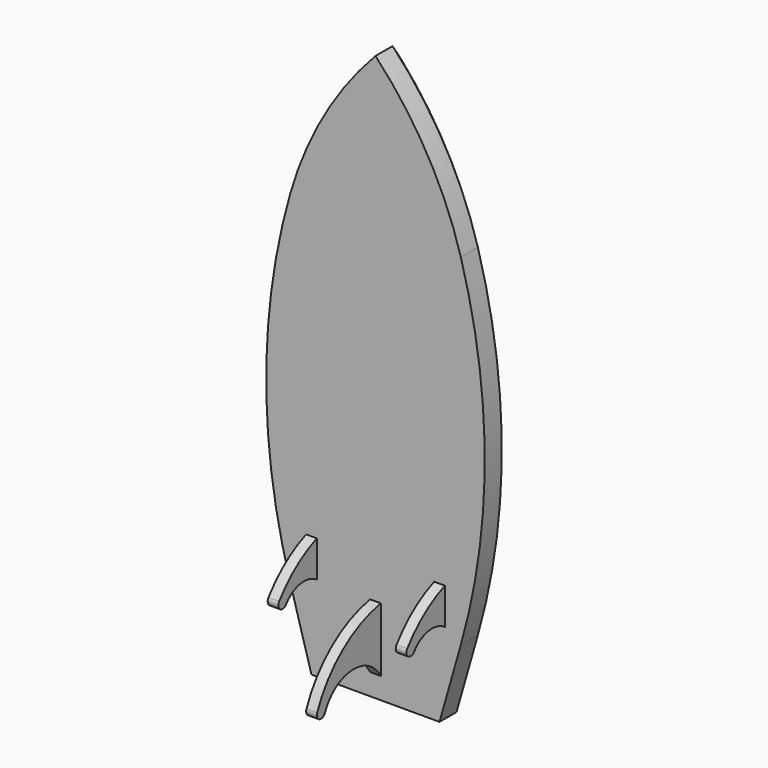
from build123d import *

# Parameters (mm, degrees)
F1_DEPTH = 4.7625
F3_DEPTH = 0.79375
F6_DEPTH = 0.79375
F7_SIZE  = 1.5875
F9_DEPTH = 1.5875


# Not quite as in the source:
# - a pattern or mirror of a feature is missing from the dataset's text; its kind, count and spacing are read off the source's solid


with BuildPart() as f1:
    # F0 (on Front) → F1 (new body)
    with BuildSketch(Plane.XZ):
        with BuildLine():
            Line((-12.7, 0), (-9.525, -11.1125))
            Line((-9.525, -11.1125), (0, -11.1125))
            Line((0, -11.1125), (9.525, -11.1125))
            Line((9.525, -11.1125), (12.7, 0))
            ThreePointArc((12.7, 0), (16.2573955939, 25.4), (12.7, 50.8))
            ThreePointArc((12.7, 50.8), (7.6947096259, 62.6809055005), (0, 73.025))
            ThreePointArc((0, 73.025), (-7.6947096259, 62.6809055005), (-12.7, 50.8))
            ThreePointArc((-12.7, 50.8), (-16.2573955939, 25.4), (-12.7, 0))
        make_face()
    extrude(amount=F1_DEPTH)

    # F2 (on Right) → F3 (join, symmetric)
    with BuildSketch(Plane.YZ):
        with BuildLine():
            Line((-4.7625, -7.9375), (-4.7625, 1.5875))
            ThreePointArc((-4.7625, 1.5875), (-11.8992437218, -1.6651672616), (-16.6078313322, -7.9375))
            ThreePointArc((-16.6078313322, -7.9375), (-16.1799545886, -8.9752859207), (-15.1421686678, -8.5474091771))
            ThreePointArc((-15.1421686678, -8.5474091771), (-10.143051775, -4.9967519132), (-4.7625, -7.9375))
        make_face()
    extrude(amount=F3_DEPTH, both=True)

    # F5 (on offset) → F6 (join, symmetric)
    with BuildSketch(Plane.YZ.offset(9.525)):
        with BuildLine():
            Line((-4.7625, 1.5875), (-4.7625, 6.9977))
            ThreePointArc((-4.7625, 6.9977), (-8.6423632972, 4.7890693745), (-11.7538487922, 1.5875))
            ThreePointArc((-11.7538487922, 1.5875), (-11.5801652534, 0.4784859544), (-10.4711512078, 0.6521694931))
            ThreePointArc((-10.4711512078, 0.6521694931), (-7.8086096464, 2.2903602428), (-4.7625, 1.5875))
        make_face()
    f6 = extrude(amount=F6_DEPTH, both=True)

    # F6_copies: F6 across plane
    add(f6.mirror(Plane(origin=(0, 0, 0), x_dir=(0, 0, -1), z_dir=(-1, 0, 0))))

    # F7
    f7_edges = [f1.edges().sort_by_distance(p)[0] for p in [
        (-16.257396, 0, 25.4),
        (16.257396, 0, 25.4),
        (0, 0, -11.1125),
        (-11.1125, 0, -5.55625),
        (11.1125, 0, -5.55625),
        (7.69471, 0, 62.680906),
        (-7.69471, 0, 62.680906),
    ]]
    chamfer(f7_edges, length=F7_SIZE)

    # F8 (on face) → F9 (cut)
    with BuildSketch(Plane(origin=(0, 0, 0), x_dir=(-1, 0, 0), z_dir=(0, 1, 0))):
        Polygon((-6.6182743758, 28.1248632818), (-6.6700917669, 25.4352521151), (4.5057865791, 25.4352521151), (4.5057865791, 28.058398515), (2.0293486305, 28.058398515), (0.9048542867, 29.1962967539), (4.5085526071, 31.6355861723), (4.5085526071, 34.4496265318), (-0.5952421925, 30.9949442744), (-3.6387769505, 33.8591597974), (-3.6387769505, 30.7964850217), (-1.2080913875, 28.5090107937), (-1.2080913875, 28.1248632818), align=None)
        with BuildLine():
            Line((0.4666208988, 17.5453214468), (-3.6424577702, 17.5453214468))
            Line((-3.6424577702, 17.5453214468), (-3.6424577702, 14.9797564372))
            Line((-3.6424577702, 14.9797564372), (0.4666208988, 14.9797564372))
            ThreePointArc((0.4666208988, 14.9797564372), (4.6440088446, 19.157144383), (0.4666208988, 23.3345323288))
            Line((0.4666208988, 23.3345323288), (-3.6424577702, 23.3345323288))
            Line((-3.6424577702, 23.3345323288), (-3.6424577702, 20.7669679075))
            Line((-3.6424577702, 20.7669679075), (0.4666208988, 20.7669679075))
            ThreePointArc((0.4666208988, 20.7669679075), (2.0774441292, 19.1561446772), (0.4666208988, 17.5453214468))
        make_face()
        with BuildLine():
            Line((8.6546270177, 44.8338016868), (6.6723674536, 44.8338016868))
            add(Edge.make_bspline(
                [(-4.5172106475, 2.828539582), (-4.2102957065, 2.1494447633), (-3.6325259568, 0.8710435159), (-2.8108192248, -0.6144651088), (-1.8892552518, -1.6043922723), (-1.0524312759, -2.1879868929), (-0.1957544902, -2.506421982), (0.7811404131, -2.2568299422), (1.5879280313, -1.7739319167), (2.1757138001, -1.1453271009), (2.6284881315, -0.4594989905), (3.409904115, 0.8193268379), (4.0612270575, 2.2527381247), (5.1265355245, 5.1336336674), (5.8584252285, 8.1588665014), (6.6285848683, 12.0725691399), (7.1356428748, 15.4950302956), (7.4330256401, 19.1136138456), (7.6363893931, 21.7933478819), (7.7823315333, 24.9471808649), (7.8520468643, 29.2726933395), (7.7372059862, 32.0576492162), (7.7120020586, 34.9143380941), (7.4839798645, 37.6447246054), (7.3090766206, 40.0269481522), (6.9398489174, 42.6509249895), (6.7587947507, 44.1284812873), (6.6723674536, 44.8338016868)],
                knots=[0, 0, 0, 0, 0.0403691258, 0.0759951914, 0.1074815982, 0.1348944717, 0.1603897512, 0.1873090479, 0.2138867667, 0.2387664663, 0.263585301, 0.2963900232, 0.3311454371, 0.3784414378, 0.4275924791, 0.4818900852, 0.5334929951, 0.5852044455, 0.629771183, 0.6785525678, 0.7354652809, 0.7815573057, 0.8274001502, 0.8726253751, 0.9150940097, 0.9594696141, 1, 1, 1, 1], degree=3))
            ThreePointArc((-4.5172106475, 2.828539582), (-5.0858860374, 2.569399443), (-5.7084131986, 2.5145793334))
            add(Edge.make_bspline(
                [(-5.7084131986, 2.5145793334), (-5.506614464, 2.0648957392), (-5.0657293675, 1.0824376715), (-3.9032511452, -0.8031134896), (-2.9635999986, -1.8497808999), (-1.9867636738, -2.5987631458), (-0.8338053387, -3.0579918443), (-0.0168141797, -3.2294336457), (0.8209716365, -3.0655957536), (1.5138835925, -2.8005151737), (2.3358805397, -2.394543116), (3.2541179547, -1.5281590897), (4.1857809915, -0.4409412593), (5.176415684, 1.2296860629), (6.2809613816, 3.4291719671), (6.9421799555, 5.2390225088), (7.6342063093, 7.5576057945), (8.099356579, 9.4090035643), (8.7001521406, 12.0174155991), (9.1556024302, 14.8338769341), (9.5981195448, 17.6634096123), (9.8314203891, 20.6701764069), (10.0211103061, 24.1869823425), (10.1148431942, 26.2740195603), (10.1813479944, 28.5970208607), (10.0793257033, 30.7502618751), (10.0643211933, 33.23997833), (9.8679121246, 36.2080072223), (9.5625129269, 39.346165649), (9.2718834561, 42.0400533513), (8.8620401687, 43.8950344105), (8.6546270177, 44.8338016868)],
                knots=[0, 0, 0, 0, 0.0307215617, 0.0671197405, 0.0962538158, 0.1231797002, 0.1502640042, 0.1725469817, 0.1946999143, 0.2157414832, 0.2389236845, 0.2662186517, 0.2954186022, 0.3296826311, 0.3680005184, 0.4024574657, 0.4400039897, 0.4741040733, 0.5138479488, 0.555501876, 0.5966862081, 0.6397342099, 0.6854696479, 0.7211558824, 0.7579160018, 0.7939211093, 0.8323591282, 0.8748241347, 0.9183554421, 0.9586813898, 1, 1, 1, 1], degree=3))
        make_face()
        with BuildLine():
            Line((0.5082425971, 38.120555704), (-3.6008360719, 38.120555704))
            Line((-3.6008360719, 38.120555704), (-3.6008360719, 35.5549906944))
            Line((-3.6008360719, 35.5549906944), (0.5082425971, 35.5549906944))
            ThreePointArc((0.5082425971, 35.5549906944), (4.6856305429, 39.7323786402), (0.5082425971, 43.909766586))
            Line((0.5082425971, 43.909766586), (-3.6008360719, 43.909766586))
            Line((-3.6008360719, 43.909766586), (-3.6008360719, 41.3422021647))
            Line((-3.6008360719, 41.3422021647), (0.5082425971, 41.3422021647))
            ThreePointArc((0.5082425971, 41.3422021647), (2.1190658274, 39.7313789343), (0.5082425971, 38.120555704))
        make_face()
        with BuildLine():
            Line((-3.6392200273, 46.105235815), (8.3869518712, 46.105235815))
            ThreePointArc((8.3869518712, 46.105235815), (8.1511000557, 47.4185871636), (7.7796555124, 48.7002059817))
            Line((7.7796555124, 48.7002059817), (4.4302197822, 48.7002059817))
            add(Edge.make_bspline(
                [(-3.6392200273, 50.0908676356), (-3.6147630306, 50.4312802898), (-3.5634048452, 51.146125879), (-2.9276489239, 52.2447330738), (-1.8123605153, 53.0774372575), (-1.022520795, 53.4070999716), (0.0082236262, 53.4837758008), (1.0487595189, 53.4282767672), (1.9530620659, 53.1404217414), (2.812366747, 52.6877708794), (3.5490772889, 51.9832733898), (4.0661254899, 51.1172716743), (4.4330181114, 50.086790062), (4.4311923281, 49.1821066237), (4.4302197822, 48.7002059817)],
                knots=[0, 0, 0, 0, 0.0818314835, 0.1718410709, 0.2660088319, 0.34016951, 0.4210124818, 0.5034808979, 0.5815208651, 0.6604699222, 0.7412360854, 0.8215356941, 0.9049368431, 1, 1, 1, 1], degree=3))
            Line((-3.6392200273, 50.0908676356), (-3.6392200273, 46.105235815))
        make_face()
        with BuildLine():
            Line((2.1111411043, 48.7319380045), (-1.4184282627, 48.7319380045))
            ThreePointArc((-1.4184282627, 48.7319380045), (0.3463564208, 51.0491565654), (2.1111411043, 48.7319380045))
        make_face(mode=Mode.SUBTRACT)
        with BuildLine():
            add(Edge.make_bspline(
                [(-8.6731268093, 12.3405372724), (-8.8621817774, 13.3043723048), (-9.2109642152, 15.082525694), (-9.4471345842, 17.0693500524), (-9.6386124998, 18.9162664816), (-9.7885706779, 20.3737065895), (-9.9207481887, 22.0261790117), (-10.0265697298, 23.9429106284), (-10.0934810707, 25.5127755009), (-10.0475649856, 27.5434312766), (-10.2027640898, 28.93724865), (-10.0617135952, 31.1767036486), (-10.0165285032, 33.0450434954), (-9.8488013785, 36.4466392996), (-9.6149967579, 38.6527351884), (-9.091986715, 42.4964440174), (-8.6370106307, 45.3946152814), (-8.0678874628, 47.9319639431), (-7.5029538136, 50.018729941), (-6.6637198417, 52.4513156556), (-6.1551610339, 53.764256506), (-5.0549762142, 56.3114139097), (-3.9287002865, 57.9396533669), (-2.5642759647, 59.3575119978), (-1.7955188836, 59.8512011078), (-1.0291619965, 60.2247262082), (-0.3305910766, 60.2683138206), (0.2312773921, 60.3188676403), (1.2576047235, 60.1260047234), (1.840494775, 59.8182049465), (2.7663610323, 59.1746101555), (3.3191036363, 58.5495702819), (3.8286805953, 57.98426908), (4.7791593797, 56.6388339733), (5.6720982961, 54.9653404882), (6.3330809754, 53.4164305846), (7.1084574097, 51.3100237545), (7.3223377778, 50.3469886777), (7.4172238819, 49.9197468162)],
                knots=[0, 0, 0, 0, 0.0355990922, 0.0656758099, 0.0942334202, 0.1198055783, 0.1470985493, 0.1763120602, 0.2033174932, 0.2330050828, 0.2585681129, 0.2894904891, 0.3193850901, 0.3577215341, 0.3902574581, 0.431511578, 0.4685019517, 0.5020949761, 0.5337761072, 0.5670910902, 0.592868579, 0.627517421, 0.6583417167, 0.6874716574, 0.7077283932, 0.7269242087, 0.7442964759, 0.7604201995, 0.7815779882, 0.7992427316, 0.8214969157, 0.840777357, 0.8589789393, 0.8860010969, 0.9153503336, 0.9432294027, 0.9748142345, 1, 1, 1, 1], degree=3))
            add(Edge.make_bspline(
                [(-8.6731268093, 12.3405372724), (-8.2762764878, 12.5553177502), (-7.5934572599, 12.9248682636), (-7.1192287591, 12.9852657111), (-6.9206189364, 13.0105605349)],
                knots=[0, 0, 0, 0, 0.5811938289, 1, 1, 1, 1], degree=3))
            add(Edge.make_bspline(
                [(-6.9206189364, 13.0105605349), (-7.0545655445, 14.1346196231), (-7.3306714156, 16.4516571201), (-7.6960844516, 20.303654636), (-7.8473616779, 24.2913940754), (-8.0014007253, 28.080079428), (-7.9002619417, 32.407236319), (-7.7558547779, 36.3221160791), (-7.3774516878, 41.0515774921), (-6.7804038779, 45.2722040082), (-5.9815007986, 49.7495152135), (-4.8592699402, 53.5352446495), (-3.8858237562, 55.7910206722), (-3.1503952318, 57.2062982168), (-2.4363002987, 58.2555137267), (-1.6527447842, 59.0112435129), (-0.9285131993, 59.506798663), (-0.2329869051, 59.6282725303), (0.7371577469, 59.5229371315), (1.3960346889, 59.1227253928), (2.0778900594, 58.5062028411), (2.8923878358, 57.3894625908), (3.8338083263, 55.6795163592), (4.6008137827, 53.5734773679), (5.289525799, 51.3872634618), (5.5747108434, 50.3729603162), (5.7021379471, 49.9197468162)],
                knots=[0, 0, 0, 0, 0.0508061154, 0.1047273009, 0.1593324972, 0.2128517735, 0.269403457, 0.3240018616, 0.3832592658, 0.4401674796, 0.498774308, 0.5533482957, 0.5959174958, 0.6300554568, 0.6606712837, 0.6892108673, 0.7143392446, 0.7371332048, 0.7637459005, 0.7875553122, 0.8133189986, 0.8452891121, 0.8835408872, 0.925064953, 0.9665173325, 1, 1, 1, 1], degree=3))
            Line((5.7021379471, 49.9197468162), (7.4172238819, 49.9197468162))
        make_face()
        with BuildLine():
            Line((-6.3328403048, 9.5369415358), (-6.7405461514, 11.8816812974))
            add(Edge.make_bspline(
                [(-6.7405461514, 11.8816812974), (-7.173686754, 11.7774624377), (-7.8419057126, 11.4846996004), (-8.589841982, 11.0327053194), (-9.0602107708, 10.5052332223), (-9.577441018, 9.746927418), (-9.7527144756, 9.0218052232), (-9.807694906, 8.2349927557), (-9.8237752096, 7.590876775), (-9.7401497586, 6.9778049775), (-9.5476026778, 6.3349817853), (-9.2236251222, 5.5720180856), (-8.76672023, 4.9932902014), (-8.2585230368, 4.5316855523), (-7.6985947623, 4.111868629), (-6.8093139027, 3.7642020371), (-5.9395215377, 3.6247698329), (-4.7865201503, 3.8050425971), (-3.9612176404, 4.1995640737), (-3.2690932586, 4.7954849), (-2.7308371531, 5.658062381), (-2.4027793571, 6.4006160688), (-2.2119444478, 7.1401437855), (-1.9716203098, 7.835301552), (-1.6059258259, 8.6069586424), (-1.3403465791, 9.1830350949), (-0.9517891163, 9.6996436765), (-0.8080399308, 9.9151184925), (-0.61323263, 10.0606255163), (-0.2820606537, 10.2399266404), (0.3142784429, 10.2279266279), (0.8448231625, 10.1383578673), (1.2940725415, 9.8493283934), (1.6470835439, 9.4795346638), (1.809165432, 9.0589124733), (1.9171228573, 8.7289977635), (2.0079113767, 7.6386792082), (1.6949066575, 6.7894305988), (1.2495667059, 6.2724815554), (0.4266842037, 5.8730657938), (-0.2050194734, 5.691374105), (-0.6107281079, 5.6296309128)],
                knots=[0, 0, 0, 0, 0.0332439606, 0.0610156138, 0.0864689022, 0.1152176349, 0.1415226571, 0.16833957, 0.1927261639, 0.2163005733, 0.2412024269, 0.2687984306, 0.2948616292, 0.3197392243, 0.3451044536, 0.3743919277, 0.4030994072, 0.4355238929, 0.4644856599, 0.4932260919, 0.5237261125, 0.5511454964, 0.577377199, 0.6035799587, 0.6314542803, 0.6561995692, 0.6802369275, 0.6954608452, 0.7098821382, 0.7281958193, 0.7515131329, 0.7738607398, 0.7957745987, 0.8174824141, 0.8372060838, 0.8551357609, 0.8864402707, 0.9154336479, 0.9398735611, 0.9681978546, 1, 1, 1, 1], degree=3))
            Line((-0.6107281079, 5.6296309128), (-0.6107281079, 3.3378668595))
            add(Edge.make_bspline(
                [(-6.3328403048, 9.5369415358), (-6.4450695538, 9.4464836666), (-6.6868975943, 9.2515679075), (-7.0958290626, 8.7971296633), (-7.2958790739, 8.2853937066), (-7.3036519657, 7.7031890487), (-7.006359204, 7.1590935954), (-6.7214102816, 6.827890977), (-6.3602314222, 6.6856091568), (-6.0679360331, 6.647423456), (-5.6954798055, 6.6836611615), (-5.3313941644, 6.9147958762), (-5.0791053594, 7.1145175505), (-4.7791838208, 7.5027349751), (-4.3350686282, 8.3200997423), (-4.0730470364, 9.1814607865), (-3.7786041771, 9.9763866455), (-3.3911365997, 10.6517965443), (-2.9084320163, 11.387910377), (-2.4565619676, 11.8392264938), (-1.7155463953, 12.4123509085), (-1.0497786054, 12.6577816233), (-0.5159951697, 12.7769650475), (-0.0302085938, 12.7754548597), (0.3642923592, 12.7888512073), (1.0590782219, 12.6554879), (1.4848236293, 12.5778132657), (1.9823193242, 12.3309977704), (2.6361048182, 12.0285135716), (3.2564256633, 11.4531883784), (3.7550531438, 10.9243468905), (4.1560758979, 10.2535718365), (4.4682347263, 9.4308294183), (4.5343393615, 8.3672221693), (4.5456701933, 7.4701050304), (4.3938809564, 6.7704256255), (4.0349513108, 5.7794370631), (3.3685568861, 4.8401773644), (2.9165748188, 4.2899691893), (2.1063190414, 3.7362307634), (1.2273621683, 3.4964893285), (0.3617214208, 3.3278300571), (-0.2808747408, 3.3344623918), (-0.6107281079, 3.3378668595)],
                knots=[0, 0, 0, 0, 0.0199979837, 0.0430910236, 0.0649956679, 0.0873337669, 0.1105384942, 0.1301227497, 0.1481491399, 0.1642268003, 0.1822078749, 0.2015504944, 0.2182139168, 0.2386665305, 0.2673673987, 0.295995366, 0.3231331983, 0.3495859868, 0.3771268596, 0.4011653057, 0.429714127, 0.4548894752, 0.4767672556, 0.4970554631, 0.5160193294, 0.5407695243, 0.5605628537, 0.5822584116, 0.607624769, 0.6349317617, 0.6603130968, 0.6862846937, 0.7141439055, 0.7449649695, 0.7729736003, 0.797866177, 0.8284472785, 0.8602759457, 0.8854692964, 0.9143746197, 0.9428444378, 0.970661271, 1, 1, 1, 1], degree=3))
        make_face()
    extrude(amount=-F9_DEPTH, mode=Mode.SUBTRACT)


solid = f1.part
